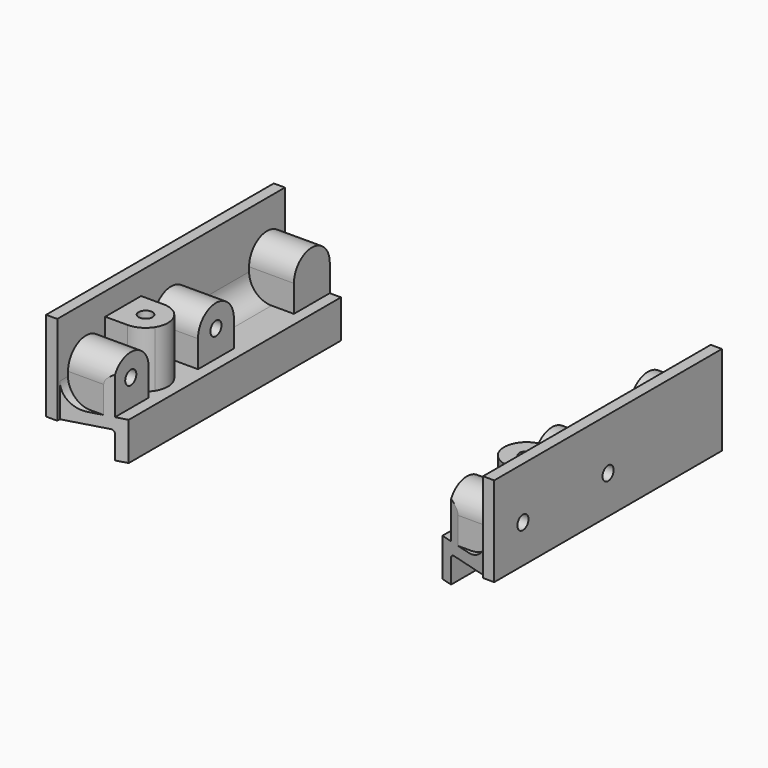
from build123d import *

# Parameters (mm, degrees)
F1_DEPTH  = 63.5
F4_DEPTH  = 25
F5_D      = 6.2
F8_DEPTH  = 30
F9_D      = 6.2
F11_DEPTH = 8
F14_DEPTH = 52.001


# Not quite as in the source:
# - a feature names something its author has since deleted; it is built from what else it names


with BuildPart() as f1:
    # F0 (on Front) → F1 (new body, symmetric)
    with BuildSketch(Plane.XZ):
        with BuildLine():
            Line((5, 40), (0, 40))
            Line((0, 40), (0, 0))
            Line((0, 0), (23.5, 0))
            ThreePointArc((23.5, 0), (24.5606601718, -0.4393398282), (25, -1.5))
            Line((25, -1.5), (25, -12))
            Line((25, -12), (30, -12))
            Line((30, -12), (30, 5))
            Line((30, 5), (15, 5))
            ThreePointArc((15, 5), (7.9289321881, 7.9289321881), (5, 15))
            Line((5, 15), (5, 40))
        make_face()
    extrude(amount=F1_DEPTH, both=True)

    # F3 (on face) → F4 (join)
    with BuildSketch(Plane(origin=(0, 0, 0), x_dir=(0, -1, 0), z_dir=(-1, 0, 0))):
        with BuildLine():
            Line((37.5, 17), (37.5, 0))
            Line((37.5, 0), (57.5, 0))
            Line((57.5, 0), (57.5, 17))
            ThreePointArc((57.5, 17), (47.5, 27), (37.5, 17))
        make_face()
        with BuildLine():
            ThreePointArc((10, 17), (0, 27), (-10, 17))
            Line((-10, 17), (-10, 0))
            Line((-10, 0), (10, 0))
            Line((10, 0), (10, 17))
        make_face()
        with BuildLine():
            Line((-63.5, 0), (-43.5, 0))
            Line((-43.5, 0), (-43.5, 17))
            ThreePointArc((-43.5, 17), (-53.5, 27), (-63.5, 17))
            Line((-63.5, 17), (-63.5, 0))
        make_face()
    extrude(amount=-F4_DEPTH)

    # F5 (through all)
    with Locations(Plane(origin=(0, 0, 0), x_dir=(0, -1, 0), z_dir=(-1, 0, 0))):
        with Locations((0, 17), (47.5, 17)):
            Hole(F5_D / 2)

    # F7 (on face) → F8 (join)
    with BuildSketch(Plane(origin=(0, 0, 0), x_dir=(1, 0, 0), z_dir=(0, 0, -1))):
        with BuildLine():
            Line((0, 16.75), (15, 16.75))
            ThreePointArc((15, 16.75), (19.8642435813, 18.0127730725), (23.5, 21.4821731236))
            Line((23.5, 21.4821731236), (23.5, 32.0178268764))
            ThreePointArc((23.5, 32.0178268764), (19.8642435813, 35.4872269275), (15, 36.75))
            Line((15, 36.75), (0, 36.75))
            Line((0, 36.75), (0, 16.75))
        make_face()
        with BuildLine():
            Line((23.5, 32.0178268764), (23.5, 21.4821731236))
            ThreePointArc((23.5, 21.4821731236), (25, 26.75), (23.5, 32.0178268764))
        make_face()
    extrude(amount=-F8_DEPTH)

    # F9 (through all)
    with Locations(Plane(origin=(0, 0, 0), x_dir=(1, 0, 0), z_dir=(0, 0, -1))):
        with Locations((15, 26.75)):
            Hole(F9_D / 2)

    # F10 (on face) → F11 (cut)
    with BuildSketch(Plane(origin=(0, 0, 0), x_dir=(1, 0, 0), z_dir=(0, 0, -1))):
        Polygon((15, 20.9764973081), (20, 23.8632486541), (20, 29.6367513459), (15, 32.5235026919), (10, 29.6367513459), (10, 23.8632486541), align=None)
    extrude(amount=-F11_DEPTH, mode=Mode.SUBTRACT)

    # F13 (on face) → F14 (cut, through all)
    with BuildSketch(Plane.XY.offset(40)):
        Polygon((40, -52.0301845696), (5, -62.0662730712), (5, -63.5), (40, -63.5), align=None)
    extrude(amount=-F14_DEPTH, mode=Mode.SUBTRACT)


with BuildPart() as f15_1:
    # F15: instance of F1
    add(f1.part.mirror(Plane.YZ.offset(100)))


solid = Compound([f1.part, f15_1.part])
